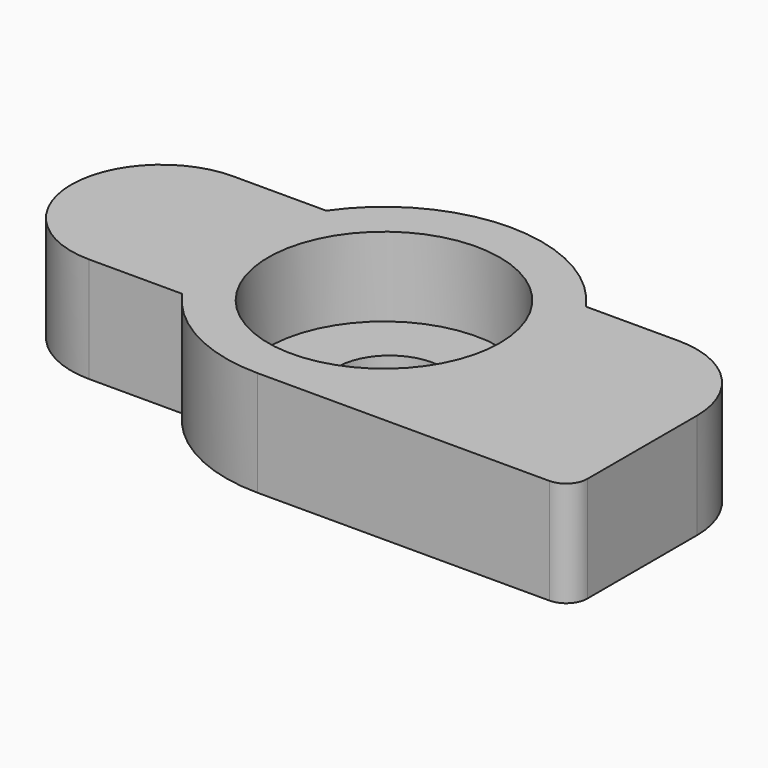
from build123d import *

# Parameters (mm, degrees)
F1_DEPTH = 10
F2_R     = 11
F3_DEPTH = 7.5
F4_R     = 4
F5_DEPTH = 7
F6_R     = 5
F7_DEPTH = 25
F8_R     = 2


# Not quite as in the source:
# - a feature names something its author has since deleted; it is built from what else it names


with BuildPart() as f1:
    # F0 (on Top) → F1 (new body)
    with BuildSketch(Plane.XY):
        with BuildLine():
            Line((29.69714, -15), (29.69714, 0))
            ThreePointArc((29.69714, 0), (27.1937406538, 6.0437406538), (21.15, 8.54714))
            Line((21.15, 8.54714), (12.3266539588, 8.54714))
            ThreePointArc((12.3266539588, 8.54714), (0, 15), (-12.3266539588, 8.54714))
            Line((-12.3266539588, 8.54714), (-21.15, 8.54714))
            ThreePointArc((-21.15, 8.54714), (-29.69714, 0), (-21.15, -8.54714))
            Line((-21.15, -8.54714), (-12.3266539588, -8.54714))
            ThreePointArc((-12.3266539588, -8.54714), (-6.9567557094, -13.2892268398), (0, -15))
            Line((0, -15), (29.69714, -15))
        make_face()
    extrude(amount=F1_DEPTH)

    # F2 (on face) → F3 (cut)
    with BuildSketch(Plane.XY.offset(10)):
        Circle(F2_R)
    extrude(amount=-F3_DEPTH, mode=Mode.SUBTRACT)

    # F4 (on face) → F5 (cut)
    with BuildSketch(Plane(origin=(0, 0, 0), x_dir=(1, 0, 0), z_dir=(0, 0, -1))):
        with Locations((-21.15, 0)):
            Circle(F4_R)
        with Locations((21.15, 0)):
            Circle(F4_R)
    extrude(amount=-F5_DEPTH, mode=Mode.SUBTRACT)

    # F6 (on face) → F7 (cut)
    with BuildSketch(Plane.XY.offset(2.5)):
        with Locations((0, 0.6768586167)):
            Circle(F6_R)
    extrude(amount=-F7_DEPTH, mode=Mode.SUBTRACT)

    # F8
    f8_edges = [f1.edges().sort_by_distance(p)[0] for p in [
        (29.69714, -15, 5),
    ]]
    fillet(f8_edges, radius=F8_R)


solid = f1.part
